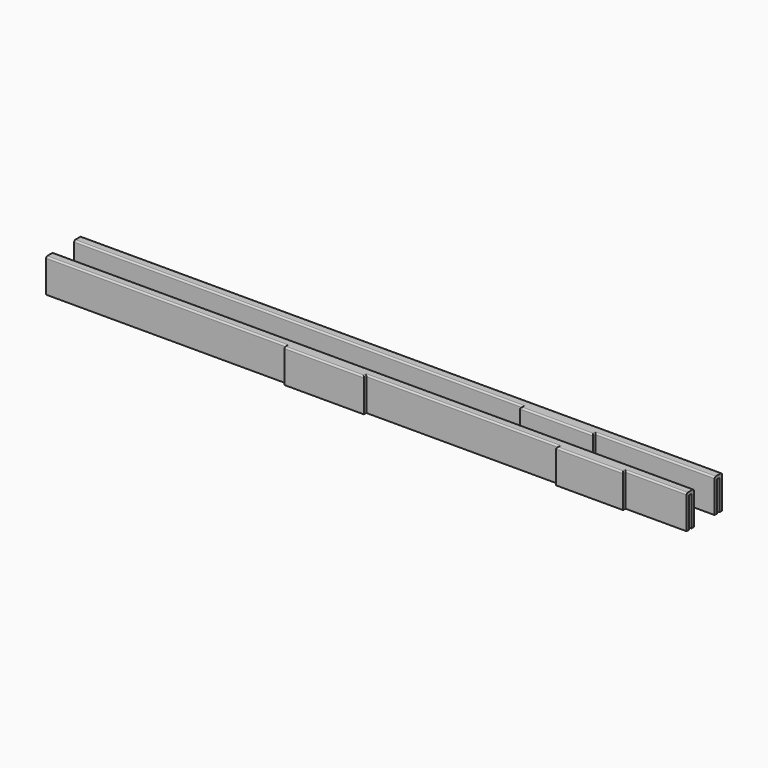
from build123d import *

# Parameters (mm, degrees)
F1_W     = 20
F1_H     = 1
F1_W_2   = 24
F2_DEPTH = 1
F1_W_3   = 210
F3_DEPTH = 11
F0_W     = 22
F0_H     = 1
F4_DEPTH = 1
F0_W_2   = 1
F0_W_3   = 210
F5_DEPTH = 11
F6_R     = 0.5
F6_2_R   = 0.5


with BuildPart() as f2:
    # F1 (on Top) → F2 (new body)
    with BuildSketch(Plane.XY):
        Polygon((105, -11), (-105, -11), (-105, -12), (-25, -12), (-1, -12), (64, -12), (84, -12), (105, -12), align=None)
        with Locations((74, -12.5)):
            Rectangle(F1_W, F1_H)
        with Locations((-13, -12.5)):
            Rectangle(F1_W_2, F1_H)
    extrude(amount=-F2_DEPTH)

    # F1 (on Top) → F3 (join)
    with BuildSketch(Plane.XY):
        with Locations((0, -10.5)):
            Rectangle(F1_W_3, F1_H)
        Polygon((-25, -13), (-26, -13), (-26, -14), (0, -14), (0, -13), (-1, -13), align=None)
        Polygon((-25, -12), (-105, -12), (-105, -13), (-26, -13), (-25, -13), align=None)
        Polygon((64, -12), (-1, -12), (-1, -13), (0, -13), (63, -13), (64, -13), align=None)
        Polygon((85, -14), (85, -13), (84, -13), (64, -13), (63, -13), (63, -14), align=None)
        Polygon((105, -13), (105, -12), (84, -12), (84, -13), (85, -13), align=None)
    extrude(amount=-F3_DEPTH)

    # F6
    f6_edges = [f2.edges().sort_by_distance(p)[0] for p in [
        (0, -10, 0),
        (-13, -14, 0),
        (0, -13.5, 0),
        (63, -13.5, 0),
        (74, -14, 0),
        (85, -13.5, 0),
        (95, -13, 0),
        (-65.5, -13, 0),
        (31.5, -13, 0),
    ]]
    fillet(f6_edges, radius=F6_R)


with BuildPart() as f4:
    # F0 (on Top) → F4 (new body)
    with BuildSketch(Plane.XY):
        Polygon((105, 0.5), (-105, 0.5), (-105, -0.5), (43, -0.5), (65, -0.5), (105, -0.5), align=None)
        with Locations((54, -1)):
            Rectangle(F0_W, F0_H)
    extrude(amount=-F4_DEPTH)

    # F0 (on Top) → F5 (join)
    with BuildSketch(Plane.XY):
        with Locations((54, -2)):
            Rectangle(F0_W, F0_H)
        with Locations((42.5, -2)):
            Rectangle(F0_W_2, F0_H)
        Polygon((43, -0.5), (-105, -0.5), (-105, -1.5), (42, -1.5), (43, -1.5), align=None)
        with Locations((65.5, -2)):
            Rectangle(F0_W_2, F0_H)
        Polygon((105, -1.5), (105, -0.5), (65, -0.5), (65, -1.5), (66, -1.5), align=None)
        with Locations((0, 1)):
            Rectangle(F0_W_3, F0_H)
    extrude(amount=-F5_DEPTH)

    # F6#2
    f6_2_edges = [f4.edges().sort_by_distance(p)[0] for p in [
        (0, 1.5, 0),
        (-31.5, -1.5, 0),
        (54, -2.5, 0),
        (85.5, -1.5, 0),
        (42, -2, 0),
        (66, -2, 0),
    ]]
    fillet(f6_2_edges, radius=F6_2_R)


solid = Compound([f2.part, f4.part])
